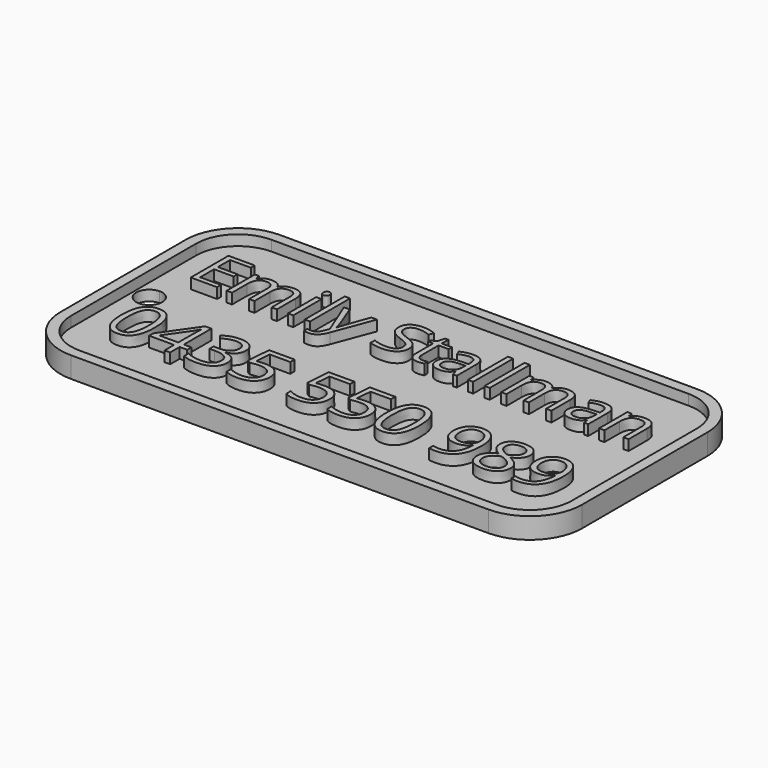
from build123d import *

# Parameters (mm, degrees)
F0_W           = 100
F0_H           = 50
F1_DEPTH       = 4
F2_T           = -2
F3_TEXT_SIZE   = 12.6392173973
F3_TEXT_SIZE_2 = 13.7641292388
F4_DEPTH       = 2
F5_R           = 8
F6_R           = 10
F8_DEPTH       = 25


# Not quite as in the source:
# - Text() gives the source's letters only with a copy of the font that has no kerning and outlines rounded to 1/6400 em; it was checked with that copy


with BuildPart() as f1:
    # F0 (on Top) → F1 (new body)
    with BuildSketch(Plane.XY):
        with Locations((-0.9568631649, -1.8714519442)):
            Rectangle(F0_W, F0_H)
    extrude(amount=F1_DEPTH)

    # F2
    f2_openings = [f1.faces().sort_by_distance(p)[0] for p in [
        (-0.956863, -1.871452, 4),
    ]]
    offset(amount=F2_T, openings=f2_openings)

    # F3 (on face) → F4 (join)
    with BuildSketch(Plane.XY.offset(2)):
        with Locations((-43.9568631649, 4.0283115297)):
            Text('Emily Stallman', F3_TEXT_SIZE, font='Open Sans', text_align=(TextAlign.LEFT, TextAlign.BOTTOM))
        with Locations((-43.9568631649, -16.8714519442)):
            Text('0435 550 989', F3_TEXT_SIZE_2, font='Open Sans', text_align=(TextAlign.LEFT, TextAlign.BOTTOM))
    extrude(amount=F4_DEPTH)

    # F5
    f5_edges = [f1.edges().sort_by_distance(p)[0] for p in [
        (47.043137, 21.128548, 3),
        (-48.956863, -24.871452, 3),
        (-48.956863, 21.128548, 3),
        (47.043137, -24.871452, 3),
    ]]
    fillet(f5_edges, radius=F5_R)

    # F6
    f6_edges = [f1.edges().sort_by_distance(p)[0] for p in [
        (-50.956863, 23.128548, 2),
        (-50.956863, -26.871452, 2),
        (49.043137, -26.871452, 2),
        (49.043137, 23.128548, 2),
    ]]
    fillet(f6_edges, radius=F6_R)

    # F7 (on face) → F8 (cut)
    with BuildSketch(Plane.XY.offset(2)):
        with BuildLine():
            ThreePointArc((-43.4568631649, -1.8714519442), (-44.1890962119, -0.1036849913), (-45.9568631649, 0.6285480558))
            Line((-45.9568631649, 0.6285480558), (-45.9568631649, -4.3714519442))
            ThreePointArc((-45.9568631649, -4.3714519442), (-44.1890962119, -3.6392188972), (-43.4568631649, -1.8714519442))
        make_face()
        with BuildLine():
            Line((-45.9568631649, -4.3714519442), (-45.9568631649, 0.6285480558))
            ThreePointArc((-45.9568631649, 0.6285480558), (-48.4568631649, -1.8714519442), (-45.9568631649, -4.3714519442))
        make_face()
    extrude(amount=-F8_DEPTH, mode=Mode.SUBTRACT)


solid = f1.part
